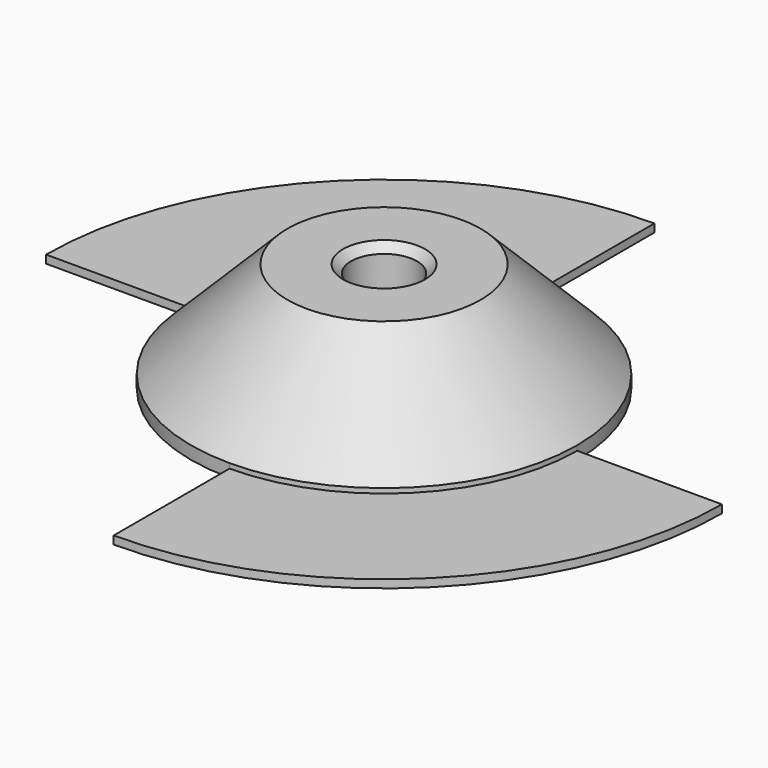
from build123d import *

# Parameters (mm, degrees)
F0_R     = 2.05
F1_DEPTH = 0.5
F2_DEPTH = 6.8
F4_SIZE  = 0.5


# Not quite as in the source:
# - a fillet or chamfer that OpenCascade refuses, or shapes differently, is made with other operations: its cross-section is extruded or revolved along the edge and cut away or added


with BuildPart() as f1:
    # F0 (on Top) → F1 (new body)
    with BuildSketch(Plane.XY):
        Circle(F0_R)
    extrude(amount=F1_DEPTH)

    # F0 (on Top) → F2 (join)
    with BuildSketch(Plane.XY):
        with BuildLine():
            ThreePointArc((0, -12), (8.4852813742, -8.4852813742), (12, 0))
            ThreePointArc((12, 0), (8.4852813742, 8.4852813742), (0, 12))
            ThreePointArc((0, 12), (-8.4852813742, 8.4852813742), (-12, 0))
            ThreePointArc((-12, 0), (-8.4852813742, -8.4852813742), (0, -12))
        make_face()
        Circle(F0_R, mode=Mode.SUBTRACT)
    extrude(amount=F2_DEPTH)

    # F3: chamfer of 6 on 1 edges, made by hand

    # F3_s1 → F3_t2 (revolve, cut)
    with BuildSketch(Plane.YZ):
        Polygon((-12, 0.8), (-6, 6.8), (-12, 6.8), align=None)
    revolve(axis=Axis((0, 0, 6.8), (0, 0, -1)), mode=Mode.SUBTRACT)

    # F4
    f4_edges = [f1.edges().sort_by_distance(p)[0] for p in [
        (-2.05, 0, 6.8),
    ]]
    chamfer(f4_edges, length=F4_SIZE)


with BuildPart() as f1b:
    # F0 (on Top) → F1, piece 2 (new body)
    with BuildSketch(Plane.XY):
        with BuildLine():
            Line((20.9999989748, -0.0065618185), (12, 0))
            ThreePointArc((12, 0), (8.4852813742, -8.4852813742), (0, -12))
            Line((0, -12), (0, -21))
            ThreePointArc((0, -21), (14.8469222705, -14.8515621769), (20.9999989748, -0.0065618185))
        make_face()
    extrude(amount=F1_DEPTH)


with BuildPart() as f1c:
    # F0 (on Top) → F1, piece 3 (new body)
    with BuildSketch(Plane.XY):
        with BuildLine():
            ThreePointArc((-12, 0), (-8.4852813742, 8.4852813742), (0, 12))
            Line((0, 12), (0, 21))
            ThreePointArc((0, 21), (-14.8492424049, 14.8492424049), (-21, 0))
            Line((-21, 0), (-12, 0))
        make_face()
    extrude(amount=F1_DEPTH)


solid = Compound([f1.part, f1b.part, f1c.part])
